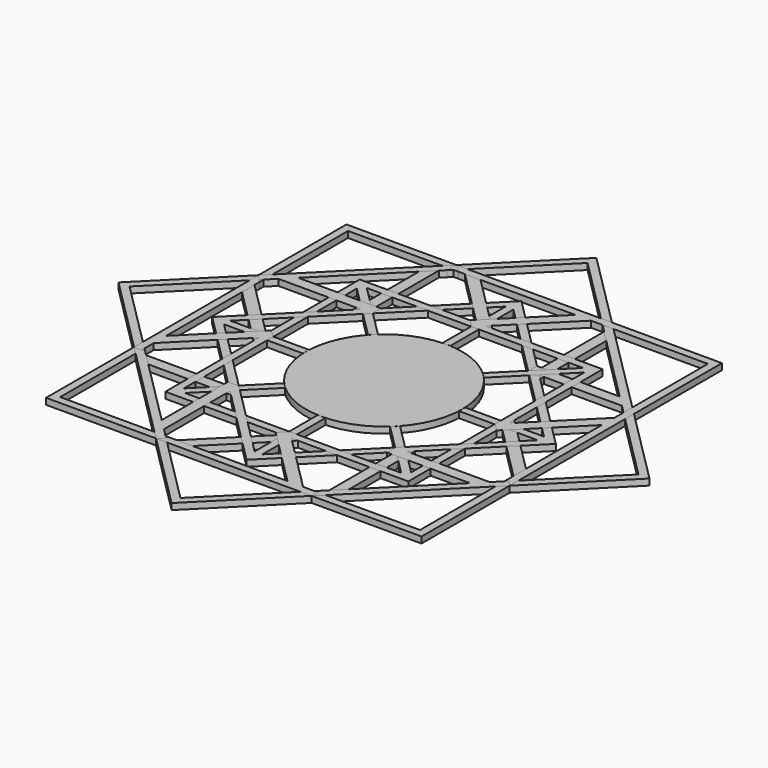
from build123d import *

# Parameters (mm, degrees)
F1_DEPTH = 2
F3_COUNT = 8


# Not quite as in the source:
# - a feature names something its author has since deleted; it is built from what else it names


with BuildPart() as f1:
    # F0 (on Top) → F1 (new body)
    with BuildSketch(Plane.XY):
        Polygon((0, 85), (0, 81.4644660941), (26.4644660941, 55), (26.4644660941, 58.5355339059), align=None)
        Polygon((26.4644660941, 55), (30, 51.4644660941), (30, 55), (26.4644660941, 58.5355339059), align=None)
        Polygon((30, 51.4644660941), (56.4644660941, 25), (60, 25), (30, 55), align=None)
        Polygon((-26.4644660941, 55), (0, 81.4644660941), (0, 85), (-26.4644660941, 58.5355339059), align=None)
        Polygon((-30, 55), (-30, 51.4644660941), (-26.4644660941, 55), (-26.4644660941, 58.5355339059), align=None)
        Polygon((-60, 25), (-56.4644660941, 25), (-30, 51.4644660941), (-30, 55), align=None)
        Polygon((-1.25, 50.2144660941), (0, 51.4644660941), (0, 55), (-26.4644660941, 28.5355339059), (-26.4644660941, 25), align=None)
        Polygon((-30, 25), (-26.4644660941, 25), (-26.4644660941, 28.5355339059), align=None)
        Polygon((0, 55), (0, 51.4644660941), (1.25, 50.2144660941), (26.4644660941, 25), (26.4644660941, 28.5355339059), align=None)
        Polygon((-30, 51.4644660941), (-30, 25), (-26.4644660941, 28.5355339059), (-26.4644660941, 55), align=None)
        Polygon((26.4644660941, 28.5355339059), (26.4644660941, 25), (30, 25), align=None)
        Polygon((26.4644660941, 28.5355339059), (30, 25), (30, 51.4644660941), (26.4644660941, 55), align=None)
        Polygon((0, 51.4644660941), (0, 25), (1.25, 25), (1.25, 50.2144660941), align=None)
        Polygon((-1.25, 25), (0, 25), (0, 51.4644660941), (-1.25, 50.2144660941), align=None)
    extrude(amount=F1_DEPTH)


with BuildPart() as f1b:
    # F0 (on Top) → F1, piece 2 (new body)
    with BuildSketch(Plane.XY):
        with BuildLine():
            ThreePointArc((-1.25, 24.9687304443), (-17.2300609401, -18.1142209327), (25, 0))
            ThreePointArc((25, 0), (18.1142209327, 17.2300609401), (1.25, 24.9687304443))
            ThreePointArc((1.25, 24.9687304443), (0.6251955264, 24.9921813885), (0, 25))
            ThreePointArc((0, 25), (-0.6251955264, 24.9921813885), (-1.25, 24.9687304443))
        make_face()
    extrude(amount=F1_DEPTH)


with BuildPart() as f3_1:
    # F3: instance of F1
    add(f1.part.rotate(Axis((0, 0, 16.1677096039), (0, 0, 1)), 1 * 360 / F3_COUNT))


with BuildPart() as f3_2:
    # F3: instance of F1
    add(f1.part.rotate(Axis((0, 0, 16.1677096039), (0, 0, 1)), 2 * 360 / F3_COUNT))


with BuildPart() as f3_3:
    # F3: instance of F1
    add(f1.part.rotate(Axis((0, 0, 16.1677096039), (0, 0, 1)), 3 * 360 / F3_COUNT))


with BuildPart() as f3_4:
    # F3: instance of F1
    add(f1.part.rotate(Axis((0, 0, 16.1677096039), (0, 0, 1)), 4 * 360 / F3_COUNT))


with BuildPart() as f3_5:
    # F3: instance of F1
    add(f1.part.rotate(Axis((0, 0, 16.1677096039), (0, 0, 1)), 5 * 360 / F3_COUNT))


with BuildPart() as f3_6:
    # F3: instance of F1
    add(f1.part.rotate(Axis((0, 0, 16.1677096039), (0, 0, 1)), 6 * 360 / F3_COUNT))


with BuildPart() as f3_7:
    # F3: instance of F1
    add(f1.part.rotate(Axis((0, 0, 16.1677096039), (0, 0, 1)), 7 * 360 / F3_COUNT))


solid = Compound([f1.part, f1b.part, f3_1.part, f3_2.part, f3_3.part, f3_4.part, f3_5.part, f3_6.part, f3_7.part])
